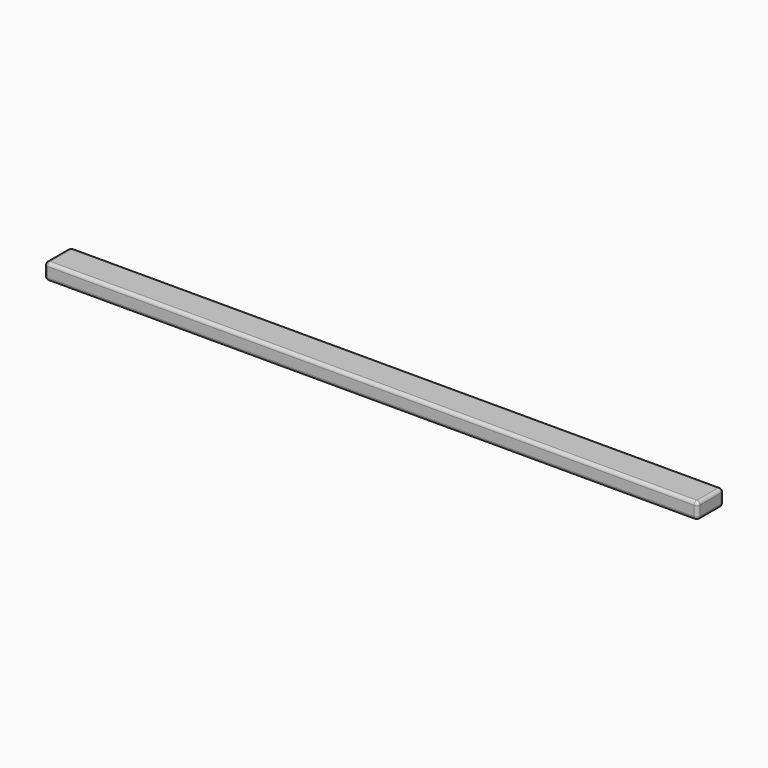
from build123d import *

# Parameters (mm, degrees)
F1_DEPTH = 1000
F2_R     = 5


with BuildPart() as f1:
    # F0 (on Right) → F1 (new body)
    with BuildSketch(Plane.YZ):
        with BuildLine():
            Line((-20, -12.5), (20, -12.5))
            ThreePointArc((20, -12.5), (23.5355339059, -11.0355339059), (25, -7.5))
            Line((25, -7.5), (25, 7.5))
            ThreePointArc((25, 7.5), (23.5355339059, 11.0355339059), (20, 12.5))
            Line((20, 12.5), (-20, 12.5))
            ThreePointArc((-20, 12.5), (-23.5355339059, 11.0355339059), (-25, 7.5))
            Line((-25, 7.5), (-25, -7.5))
            ThreePointArc((-25, -7.5), (-23.5355339059, -11.0355339059), (-20, -12.5))
        make_face()
    extrude(amount=F1_DEPTH)

    # F2
    f2_edges = [f1.edges().sort_by_distance(p)[0] for p in [
        (1000, -25, 0),
        (0, 25, 0),
    ]]
    fillet(f2_edges, radius=F2_R)


solid = f1.part
